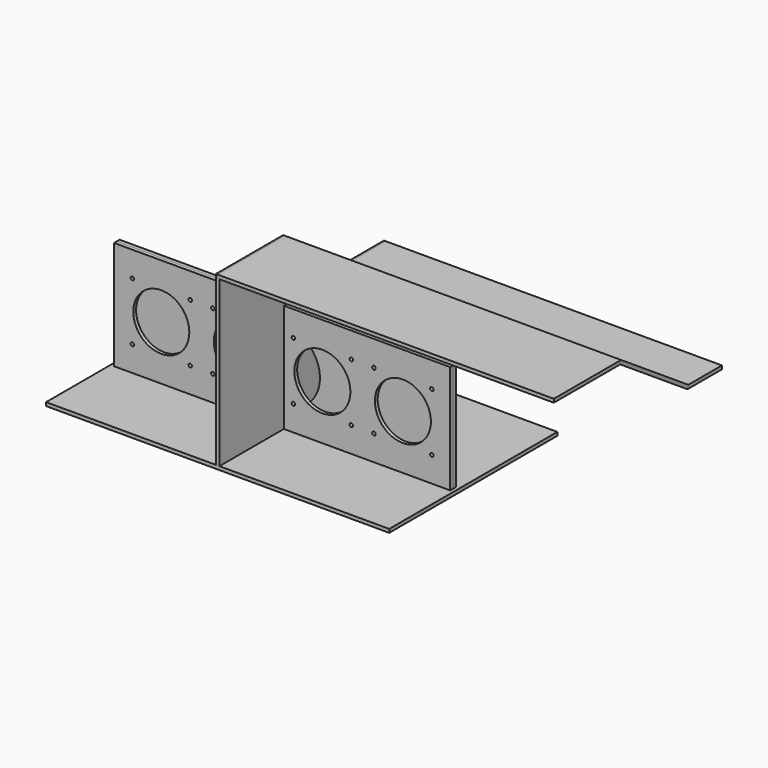
from build123d import *

# Parameters (mm, degrees)
F1_DEPTH = 3.175
F2_W     = 622.3
F2_H     = 381
F3_DEPTH = 6.35
F4_W     = 609.6
F4_H     = 196.85
F4_R     = 50.8
F5_DEPTH = 6.35
F6_DEPTH = 609.6
F7_DEPTH = 609.6
F8_DEPTH = 609.6
F9_DEPTH = 6.35
F10_D    = 6.35


# Not quite as in the source:
# - a feature names something its author has since deleted; it is built from what else it names


with BuildPart() as f1:
    # F0 (on Right) → F1 (new body, symmetric)
    with BuildSketch(Plane.YZ):
        Polygon((-152.4, 298.45), (-152.4, 0), (228.6, 0), (228.6, 196.85), (150.4773747004, 196.85), (-1.9226252996, 298.45), align=None)
        Polygon((150.4773747004, 196.85), (228.6, 196.85), (228.6, 203.2), (152.4, 203.2), align=None)
        Polygon((0, 304.8), (-1.9226252996, 298.45), (150.4773747004, 196.85), (152.4, 203.2), align=None)
        Polygon((-152.4, 304.8), (-152.4, 298.45), (-1.9226252996, 298.45), (0, 304.8), align=None)
    extrude(amount=F1_DEPTH, both=True)


with BuildPart() as f3:
    # F2 (on Top) → F3 (new body)
    with BuildSketch(Plane.XY):
        with Locations((0, 38.1)):
            Rectangle(F2_W, F2_H)
    extrude(amount=-F3_DEPTH)


with BuildPart() as f5:
    # F4 (on Front) → F5 (new body)
    with BuildSketch(Plane.XZ):
        with Locations((0, 98.425)):
            Rectangle(F4_W, F4_H)
        with Locations((-219.075, 98.425)):
            Circle(F4_R, mode=Mode.SUBTRACT)
        with BuildLine():
            ThreePointArc((-46.4516304348, 55.1295495467), (-123.825, 98.425), (-46.4516304348, 141.7204504533))
            ThreePointArc((-46.4516304348, 141.7204504533), (0, 161.925), (46.4516304348, 141.7204504533))
            ThreePointArc((46.4516304348, 141.7204504533), (97.831378475, 142.756519114), (123.825, 98.425))
            ThreePointArc((123.825, 98.425), (97.831378475, 54.093480886), (46.4516304348, 55.1295495467))
            ThreePointArc((46.4516304348, 55.1295495467), (0, 34.925), (-46.4516304348, 55.1295495467))
        make_face(mode=Mode.SUBTRACT)
        with Locations((219.075, 98.425)):
            Circle(F4_R, mode=Mode.SUBTRACT)
        with Locations((-219.075, 98.425)):
            Circle(F4_R)
        with Locations((219.075, 98.425)):
            Circle(F4_R)
        with BuildLine():
            ThreePointArc((-46.4516304348, 55.1295495467), (-63.5, 98.425), (-46.4516304348, 141.7204504533))
            ThreePointArc((-46.4516304348, 141.7204504533), (-123.825, 98.425), (-46.4516304348, 55.1295495467))
        make_face()
        with BuildLine():
            ThreePointArc((123.825, 98.425), (97.831378475, 142.756519114), (46.4516304348, 141.7204504533))
            ThreePointArc((46.4516304348, 141.7204504533), (59.0843825922, 121.690548214), (63.5, 98.425))
            ThreePointArc((63.5, 98.425), (59.0843825922, 75.159451786), (46.4516304348, 55.1295495467))
            ThreePointArc((46.4516304348, 55.1295495467), (97.831378475, 54.093480886), (123.825, 98.425))
        make_face()
    extrude(amount=-F5_DEPTH)


with BuildPart() as f6:
    # F0 (on Right) → F6 (new body)
    with BuildSketch(Plane.YZ):
        Polygon((-152.4, 304.8), (-152.4, 298.45), (-1.9226252996, 298.45), (0, 304.8), align=None)
    extrude(amount=F6_DEPTH)


with BuildPart() as f7:
    # F0 (on Right) → F7 (new body)
    with BuildSketch(Plane.YZ):
        Polygon((0, 304.8), (-1.9226252996, 298.45), (150.4773747004, 196.85), (152.4, 203.2), align=None)
    extrude(amount=F7_DEPTH)


with BuildPart() as f8:
    # F0 (on Right) → F8 (new body)
    with BuildSketch(Plane.YZ):
        Polygon((150.4773747004, 196.85), (228.6, 196.85), (228.6, 203.2), (152.4, 203.2), align=None)
    extrude(amount=F8_DEPTH)


with BuildPart() as f9:
    # F4 (on Front) → F9 (new body)
    with BuildSketch(Plane.XZ):
        with Locations((0, 98.425)):
            Rectangle(F4_W, F4_H)
        with Locations((-219.075, 98.425)):
            Circle(F4_R, mode=Mode.SUBTRACT)
        with BuildLine():
            ThreePointArc((-46.4516304348, 55.1295495467), (-123.825, 98.425), (-46.4516304348, 141.7204504533))
            ThreePointArc((-46.4516304348, 141.7204504533), (0, 161.925), (46.4516304348, 141.7204504533))
            ThreePointArc((46.4516304348, 141.7204504533), (97.831378475, 142.756519114), (123.825, 98.425))
            ThreePointArc((123.825, 98.425), (97.831378475, 54.093480886), (46.4516304348, 55.1295495467))
            ThreePointArc((46.4516304348, 55.1295495467), (0, 34.925), (-46.4516304348, 55.1295495467))
        make_face(mode=Mode.SUBTRACT)
        with Locations((219.075, 98.425)):
            Circle(F4_R, mode=Mode.SUBTRACT)
        with BuildLine():
            ThreePointArc((-46.4516304348, 141.7204504533), (-28.693480886, 123.231378475), (-22.225, 98.425))
            ThreePointArc((-22.225, 98.425), (-28.693480886, 73.618621525), (-46.4516304348, 55.1295495467))
            ThreePointArc((-46.4516304348, 55.1295495467), (0, 34.925), (46.4516304348, 55.1295495467))
            ThreePointArc((46.4516304348, 55.1295495467), (22.225, 98.425), (46.4516304348, 141.7204504533))
            ThreePointArc((46.4516304348, 141.7204504533), (0, 161.925), (-46.4516304348, 141.7204504533))
        make_face()
    extrude(amount=F9_DEPTH)

    # F10 (through all)
    with Locations(Plane(origin=(0, 0, 0), x_dir=(1, 0, 0), z_dir=(0, 1, 0))):
        with Locations((-271.575, -150.925), (-166.575, -150.925), (-125.525, -150.925), (-125.525, -45.925), (-166.575, -45.925), (-271.575, -45.925), (-20.525, -150.925), (20.525, -150.925), (-20.525, -45.925), (20.525, -45.925), (125.525, -150.925), (166.575, -150.925), (271.575, -150.925), (271.575, -45.925), (166.575, -45.925), (125.525, -45.925)):
            Hole(F10_D / 2)


solid = Compound([f1.part, f3.part, f5.part, f6.part, f7.part, f8.part, f9.part])
